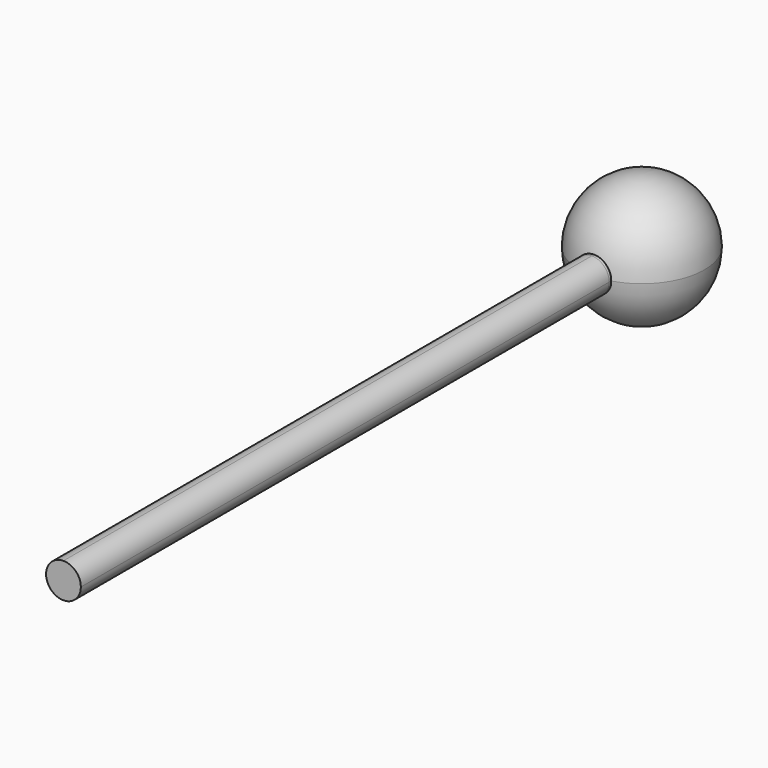
from build123d import *

# Parameters (mm, degrees)
F1_DEPTH = 95
F5_DEPTH = 0.5


with BuildPart() as f1:
    # F0 (on Front) → F1 (new body)
    with BuildSketch(Plane.XZ):
        with BuildLine():
            Line((0, -2.5), (0, 2.5))
            ThreePointArc((0, 2.5), (-2.5, 0), (0, -2.5))
        make_face()
        with BuildLine():
            ThreePointArc((0, -2.5), (1.767766953, -1.767766953), (2.5, 0))
            ThreePointArc((2.5, 0), (1.767766953, 1.767766953), (0, 2.5))
            Line((0, 2.5), (0, -2.5))
        make_face()
    extrude(amount=F1_DEPTH)


with BuildPart() as f4:
    # F3 (on face) → F4 (revolve)
    with BuildSketch(Plane.YZ):
        with BuildLine():
            ThreePointArc((9, -9), (15.3639610307, -6.3639610307), (18, 0))
            ThreePointArc((18, 0), (15.3639610307, 6.3639610307), (9, 9))
            Line((9, 9), (9, 2.5))
            Line((9, 2.5), (9, 0))
            Line((9, 0), (9, -2.5))
            Line((9, -2.5), (9, -9))
        make_face()
    revolve(axis=Axis((0, 9, 0), (0, 0, -1)))


with BuildPart() as f5:
    # F5 (new): a face of the model
    f5_faces = [f1.part.faces().sort_by_distance(p)[0] for p in [
        (0, 0, 0),
    ]]
    extrude(f5_faces, amount=F5_DEPTH)


solid = Compound([f1.part, f4.part, f5.part])
